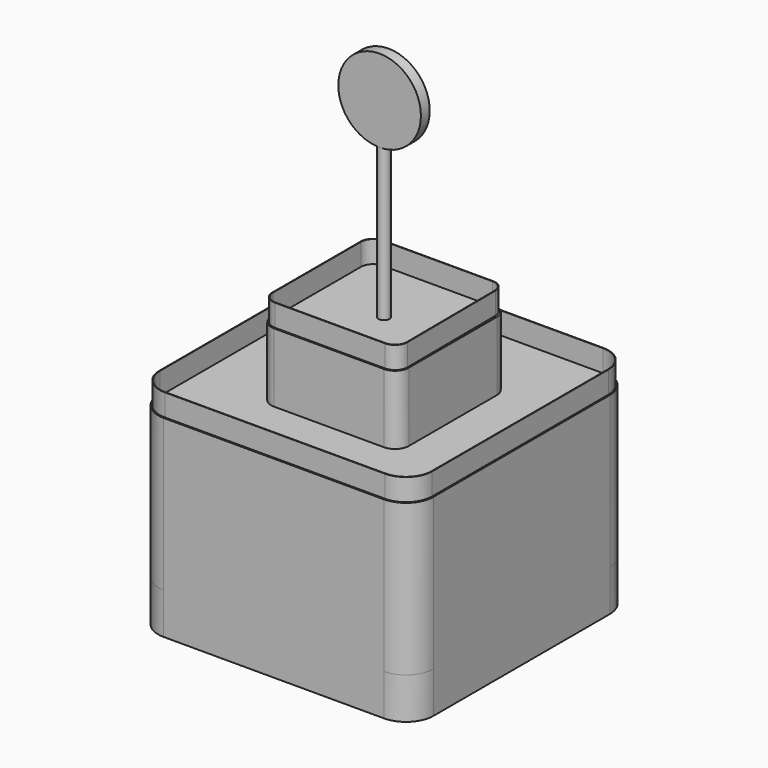
from build123d import *

# Parameters (mm, degrees)
F2_W      = 900
F2_H      = 900
F3_DEPTH  = 150
F4_W      = 1000
F4_H      = 1000
F5_DEPTH  = 550
F6_W      = 500
F6_H      = 500
F7_DEPTH  = 250
F8_R      = 100
F9_R      = 85
F10_R     = 50
F12_DEPTH = 80
F14_DEPTH = 80
F15_R     = 20
F16_DEPTH = 1600
F18_R     = 150
F19_DEPTH = 20
F21_DEPTH = 150


# Not quite as in the source:
# - a feature of the source that left no trace in its solid (it failed there, or was rolled back) is left out


with BuildPart() as f3:
    # F2 (on Top) → F3 (new body, through all)
    with BuildSketch(Plane.XY):
        Rectangle(F2_W, F2_H)
    extrude(amount=F3_DEPTH)

    # F4 (on face) → F5 (join, through all)
    with BuildSketch(Plane.XY.offset(150)):
        Rectangle(F4_W, F4_H)
    extrude(amount=F5_DEPTH)

    # F6 (on face) → F7 (join)
    with BuildSketch(Plane.XY.offset(700)):
        Rectangle(F6_W, F6_H)
    extrude(amount=F7_DEPTH)

    # F8
    f8_edges = [f3.edges().sort_by_distance(p)[0] for p in [
        (500, -500, 425),
        (-500, -500, 425),
        (500, 500, 425),
        (-500, 500, 425),
    ]]
    fillet(f8_edges, radius=F8_R)

    # F9
    f9_edges = [f3.edges().sort_by_distance(p)[0] for p in [
        (-450, 450, 75),
        (-450, -450, 75),
        (450, -450, 75),
        (450, 450, 75),
    ]]
    fillet(f9_edges, radius=F9_R)

    # F10
    f10_edges = [f3.edges().sort_by_distance(p)[0] for p in [
        (-250, -250, 825),
        (250, -250, 825),
        (250, 250, 825),
        (-250, 250, 825),
    ]]
    fillet(f10_edges, radius=F10_R)

    # F15 (on Top) → F16 (join)
    with BuildSketch(Plane.XY):
        Circle(F15_R)
    extrude(amount=F16_DEPTH)

    # F18 (on Front) → F19 (join, symmetric)
    with BuildSketch(Plane.XZ):
        with Locations((0, 1650)):
            Circle(F18_R)
    extrude(amount=F19_DEPTH, both=True)

    # F20 (on face) → F21 (join, through all)
    with BuildSketch(Plane(origin=(0, 0, 150), x_dir=(1, 0, 0), z_dir=(0, 0, -1))):
        with BuildLine():
            Line((400, 500), (-400, 500))
            ThreePointArc((-400, 500), (-470.7106781187, 470.7106781187), (-500, 400))
            Line((-500, 400), (-500, -400))
            ThreePointArc((-500, -400), (-470.7106781187, -470.7106781187), (-400, -500))
            Line((-400, -500), (400, -500))
            ThreePointArc((400, -500), (470.7106781187, -470.7106781187), (500, -400))
            Line((500, -400), (500, 400))
            ThreePointArc((500, 400), (470.7106781187, 470.7106781187), (400, 500))
        make_face()
        with BuildLine():
            ThreePointArc((365, 450), (425.1040764009, 425.1040764009), (450, 365))
            Line((450, 365), (450, -365))
            ThreePointArc((450, -365), (425.1040764009, -425.1040764009), (365, -450))
            Line((365, -450), (-365, -450))
            ThreePointArc((-365, -450), (-425.1040764009, -425.1040764009), (-450, -365))
            Line((-450, -365), (-450, 365))
            ThreePointArc((-450, 365), (-425.1040764009, 425.1040764009), (-365, 450))
            Line((-365, 450), (365, 450))
        make_face(mode=Mode.SUBTRACT)
    extrude(amount=F21_DEPTH)


with BuildPart() as f12:
    # F11 (on face) → F12 (new body)
    with BuildSketch(Plane.XY.offset(700)):
        with BuildLine():
            ThreePointArc((-400, 495), (-467.1751442127, 467.1751442127), (-495, 400))
            Line((-495, 400), (-495, -400))
            ThreePointArc((-495, -400), (-467.1751442127, -467.1751442127), (-400, -495))
            Line((-400, -495), (400, -495))
            ThreePointArc((400, -495), (467.1751442127, -467.1751442127), (495, -400))
            Line((495, -400), (495, 400))
            ThreePointArc((495, 400), (467.1751442127, 467.1751442127), (400, 495))
            Line((400, 495), (-400, 495))
        make_face()
        with BuildLine():
            ThreePointArc((493, -400), (465.7609306503, -465.7609306503), (400, -493))
            Line((400, -493), (-400, -493))
            ThreePointArc((-400, -493), (-465.7609306503, -465.7609306503), (-493, -400))
            Line((-493, -400), (-493, 400))
            ThreePointArc((-493, 400), (-465.7609306503, 465.7609306503), (-400, 493))
            Line((-400, 493), (400, 493))
            ThreePointArc((400, 493), (465.7609306503, 465.7609306503), (493, 400))
            Line((493, 400), (493, -400))
        make_face(mode=Mode.SUBTRACT)
    extrude(amount=F12_DEPTH)


with BuildPart() as f14:
    # F13 (on face) → F14 (new body)
    with BuildSketch(Plane.XY.offset(950)):
        with BuildLine():
            ThreePointArc((242.0000088609, 203.0075300193), (229.6958274631, 232.7011505768), (200, 245.0000047089))
            Line((200, 245.0000047089), (-200, 245.0000047089))
            ThreePointArc((-200, 245.0000047089), (-231.8198084831, 231.8198084831), (-245.0000047089, 200))
            Line((-245.0000047089, 200), (-245.0000047089, -200))
            ThreePointArc((-245.0000047089, -200), (-231.8198084831, -231.8198084831), (-200, -245.0000047089))
            Line((-200, -245.0000047089), (200, -245.0000047089))
            ThreePointArc((200, -245.0000047089), (232.0531499414, -231.5847431942), (244.9951290454, -199.3375907688))
            Line((244.9951290454, -199.3375907688), (242.0000088609, 203.0075300193))
        make_face()
        with BuildLine():
            ThreePointArc((-243.0000047089, 200), (-230.4055949208, 230.4055949208), (-200, 243.0000047089))
            Line((-200, 243.0000047089), (200, 243.0000047089))
            ThreePointArc((200, 243.0000047089), (228.284277991, 231.2842731632), (240.0000095367, 202.9999951722))
            Line((240.0000095367, 202.9999951722), (243.0000047089, -200))
            ThreePointArc((243.0000047089, -200), (230.4055949208, -230.4055949208), (200, -243.0000047089))
            Line((200, -243.0000047089), (-200, -243.0000047089))
            ThreePointArc((-200, -243.0000047089), (-230.4055949208, -230.4055949208), (-243.0000047089, -200))
            Line((-243.0000047089, -200), (-243.0000047089, 200))
        make_face(mode=Mode.SUBTRACT)
    extrude(amount=F14_DEPTH)


solid = Compound([f3.part, f12.part, f14.part])
